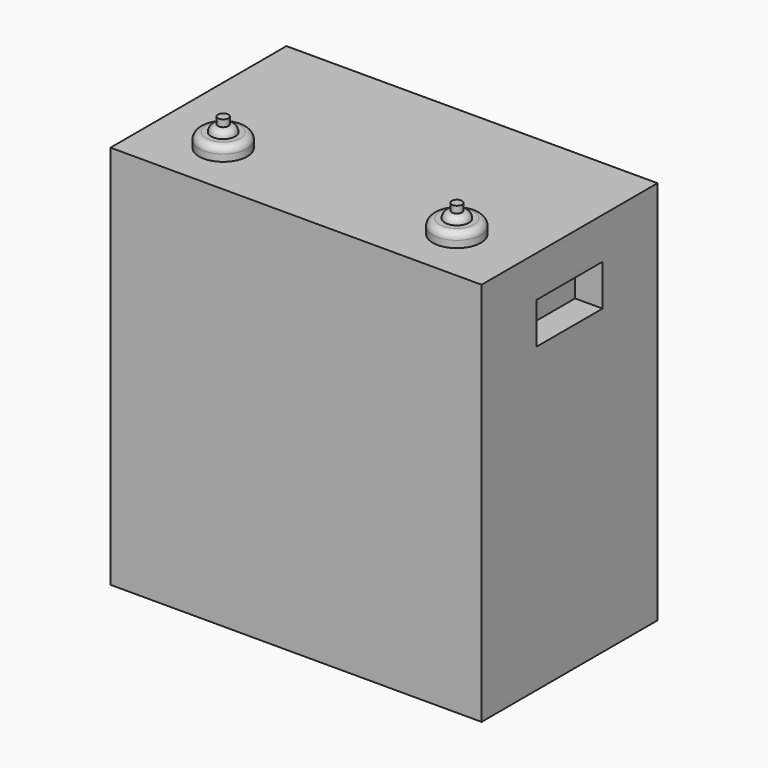
from build123d import *

# Parameters (mm, degrees)
F0_W     = 342.9
F0_H     = 203.2
F1_DEPTH = 355.6
F6_W     = 76.2
F6_H     = 38.1
F7_DEPTH = 25.4


# Not quite as in the source:
# - a pattern or mirror of a feature is missing from the dataset's text; its kind, count and spacing are read off the source's solid


with BuildPart() as f1:
    # F0 (on Top) → F1 (new body)
    with BuildSketch(Plane.XY):
        with Locations((171.45, 101.6)):
            Rectangle(F0_W, F0_H)
    extrude(amount=F1_DEPTH)

    # F3 (on offset) → F4 (revolve)
    with BuildSketch(Plane.XZ.offset(-50.8)):
        with BuildLine():
            Line((63.5, 381), (63.5, 355.6))
            Line((63.5, 355.6), (85.725, 355.6))
            Line((85.725, 355.6), (85.725, 361.95))
            ThreePointArc((85.725, 361.95), (83.8651280605, 366.4401280605), (79.375, 368.3))
            Line((79.375, 368.3), (74.6125, 368.3))
            ThreePointArc((74.6125, 368.3), (72.7526280605, 372.7901280605), (68.2625, 374.65))
            Line((68.2625, 374.65), (68.2625, 381))
            Line((68.2625, 381), (63.5, 381))
        make_face()
    f4 = revolve(axis=Axis((63.5, 50.8, 362.4166101217), (0, 0, 1)))

    # F4_copies: F4 across plane
    add(f4.mirror(Plane(origin=(171.45, 0, 0), x_dir=(0, 0, 1), z_dir=(1, 0, 0))))

    # F6 (on face) → F7 (cut)
    with BuildSketch(Plane(origin=(0, 0, 0), x_dir=(0, -1, 0), z_dir=(-1, 0, 0))):
        with Locations((-101.6, 298.45)):
            Rectangle(F6_W, F6_H)
    f7 = extrude(amount=-F7_DEPTH, mode=Mode.SUBTRACT)

    # F7_copies: F7 across plane
    add(f7.mirror(Plane(origin=(171.45, 0, 0), x_dir=(0, 0, 1), z_dir=(1, 0, 0))), mode=Mode.SUBTRACT)


solid = f1.part
